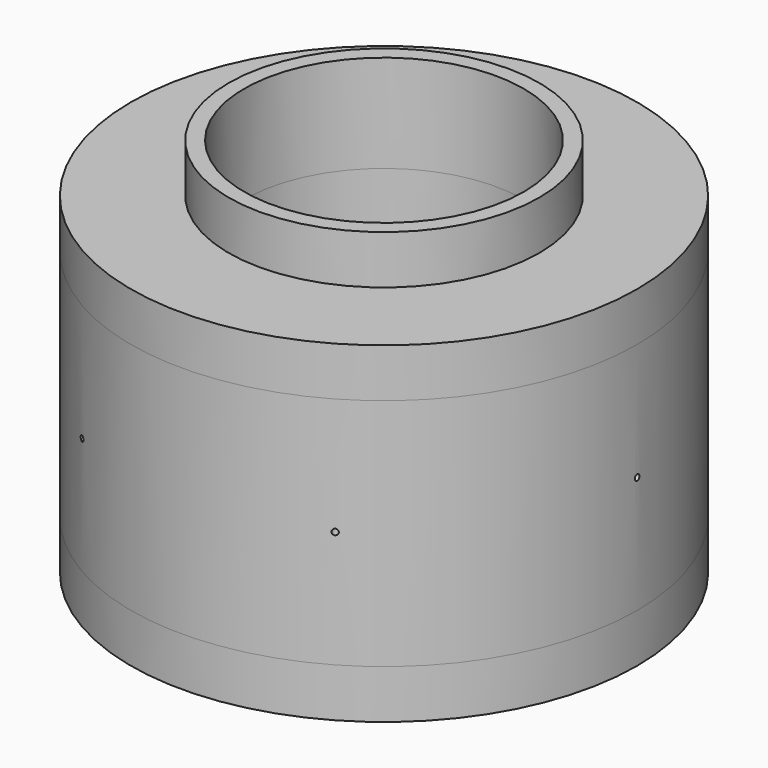
from build123d import *

# Parameters (mm, degrees)
F0_R             = 129.775
F1_DEPTH         = 25
F2_R             = 79.62
F3_DEPTH         = 25
F4_R             = 71.655
F5_DEPTH         = 50
F6_R             = 129.775
F7_DEPTH         = 120
F9_DEPTH         = 170.001
F8_R             = 1.5
F10_DEPTH        = 129.776
F10_COPIES_COUNT = 6


# Not quite as in the source:
# - a pattern or mirror of a feature is missing from the dataset's text; its kind, count and spacing are read off the source's solid


with BuildPart() as f1:
    # F0 (on Top) → F1 (new body)
    with BuildSketch(Plane.XY):
        Circle(F0_R)
    extrude(amount=F1_DEPTH)

    # F2 (on face) → F3 (join)
    with BuildSketch(Plane.XY.offset(25)):
        Circle(F2_R)
    extrude(amount=F3_DEPTH)

    # F4 (on face) → F5 (cut, through all)
    with BuildSketch(Plane.XY.offset(50)):
        Circle(F4_R)
    extrude(amount=-F5_DEPTH, mode=Mode.SUBTRACT)


with BuildPart() as f7:
    # F6 (on Top) → F7 (new body)
    with BuildSketch(Plane.XY):
        Circle(F6_R)
    extrude(amount=-F7_DEPTH)

    # F4 (on face) → F9 (cut, through all)
    with BuildSketch(Plane.XY.offset(50)):
        Circle(F4_R)
    extrude(amount=-F9_DEPTH, mode=Mode.SUBTRACT)

    # F8 (on Right) → F10 (cut, through all)
    with BuildSketch(Plane.YZ):
        with Locations((0, -60)):
            Circle(F8_R)
    f10 = extrude(amount=-F10_DEPTH, mode=Mode.SUBTRACT)

    # F10_copies: F10 ×6 about axis
    f10_copies_axis = Axis((0, 0, 0), (0, 0, 1))
    for i in range(1, F10_COPIES_COUNT):
        add(f10.rotate(f10_copies_axis, i * 360 / F10_COPIES_COUNT), mode=Mode.SUBTRACT)


with BuildPart() as f12_1:
    # F12: instance of F1
    add(f1.part.mirror(Plane.XY.offset(-60)))


solid = Compound([f1.part, f7.part, f12_1.part])
